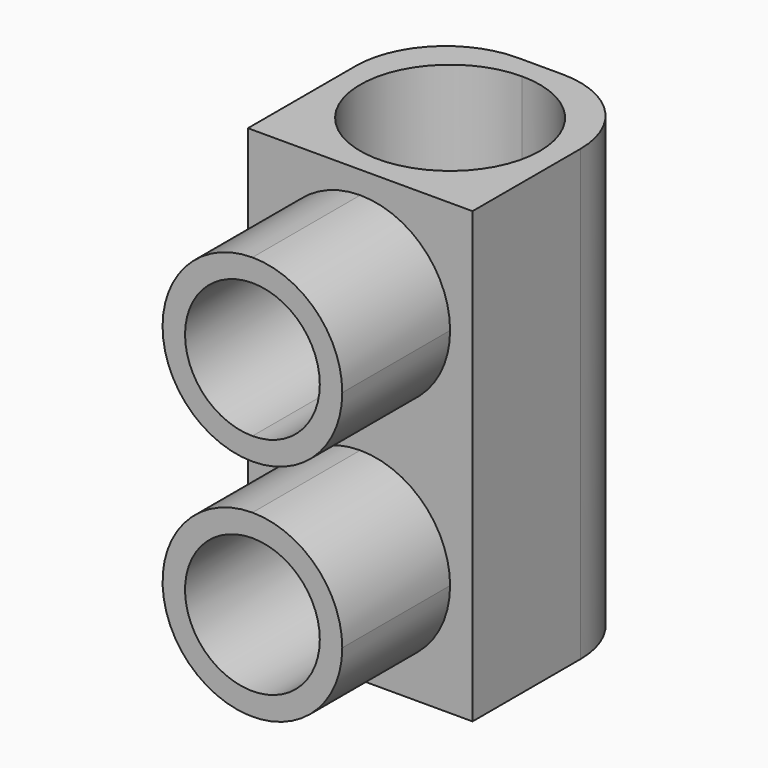
from build123d import *

# Parameters (mm, degrees)
F0_W      = 5
F0_H      = 10
F1_DEPTH  = 4
F2_W      = 2
F2_H      = 4
F3_DEPTH  = 25
F4_R      = 2
F7_DEPTH  = 3
F8_DEPTH  = 25
F9_R      = 1
F10_DEPTH = 2


# Not quite as in the source:
# - a feature names something its author has since deleted; it is built from what else it names


with BuildPart() as f1:
    # F0 (on Front) → F1 (new body, symmetric)
    with BuildSketch(Plane.XZ):
        Rectangle(F0_W, F0_H)
    extrude(amount=F1_DEPTH, both=True)

    # F2 (on face) → F3 (cut)
    with BuildSketch(Plane.XZ.offset(4)):
        with Locations((3.5, 3)):
            Rectangle(F2_W, F2_H)
        with Locations((10.5, 3)):
            Rectangle(F2_W, F2_H)
        with Locations((17.5, 3)):
            Rectangle(F2_W, F2_H)
        with Locations((17.5, -3)):
            Rectangle(F2_W, F2_H)
        with Locations((10.5, -3)):
            Rectangle(F2_W, F2_H)
        with Locations((3.5, -3)):
            Rectangle(F2_W, F2_H)
    extrude(amount=-F3_DEPTH, mode=Mode.SUBTRACT)

    # F4
    f4_edges = [f1.edges().sort_by_distance(p)[0] for p in [
        (-2.5, 4, 0),
        (2.5, 4, 0),
    ]]
    fillet(f4_edges, radius=F4_R)

    # F6 (on face) → F7 (cut)
    with BuildSketch(Plane.XZ.offset(4)):
        Polygon((2.5, 5), (0, 5), (-2.5, 5), (-2.5, -5), (2.5, -5), align=None)
        with BuildLine():
            ThreePointArc((2, -2.5), (-1.4142135624, -3.9142135624), (0, -0.5))
            ThreePointArc((0, -0.5), (1.4142135624, -1.0857864376), (2, -2.5))
        make_face(mode=Mode.SUBTRACT)
        with BuildLine():
            ThreePointArc((0, 0.5), (-2, 2.5), (0, 4.5))
            ThreePointArc((0, 4.5), (1.4142135624, 3.9142135624), (2, 2.5))
            ThreePointArc((2, 2.5), (1.4142135624, 1.0857864376), (0, 0.5))
        make_face(mode=Mode.SUBTRACT)
        with BuildLine():
            ThreePointArc((1.5, -2.5), (1.0606601718, -1.4393398282), (0, -1))
            ThreePointArc((0, -1), (-1.0606601718, -3.5606601718), (1.5, -2.5))
        make_face()
        with BuildLine():
            Line((0, 2.5), (0, 4))
            ThreePointArc((0, 4), (-1.5, 2.5), (0, 1))
            Line((0, 1), (0, 2.5))
        make_face()
        with BuildLine():
            ThreePointArc((1.5, 2.5), (1.0606601718, 3.5606601718), (0, 4))
            Line((0, 4), (0, 2.5))
            Line((0, 2.5), (0, 1))
            ThreePointArc((0, 1), (1.0606601718, 1.4393398282), (1.5, 2.5))
        make_face()
    extrude(amount=-F7_DEPTH, mode=Mode.SUBTRACT)

    # F5 (on face) → F8 (cut)
    with BuildSketch(Plane.XY.offset(5)):
        with BuildLine():
            ThreePointArc((2, 1.5), (1.4142135624, 2.9142135624), (0, 3.5))
            ThreePointArc((0, 3.5), (-1.4142135624, 0.0857864376), (2, 1.5))
        make_face()
    extrude(amount=-F8_DEPTH, mode=Mode.SUBTRACT)

    # F9 (on face) → F10 (join)
    with BuildSketch(Plane(origin=(-2.5, 0, 0), x_dir=(0, -1, 0), z_dir=(-1, 0, 0))):
        with Locations((-0.5, 0)):
            Circle(F9_R)
    extrude(amount=F10_DEPTH)


solid = f1.part
